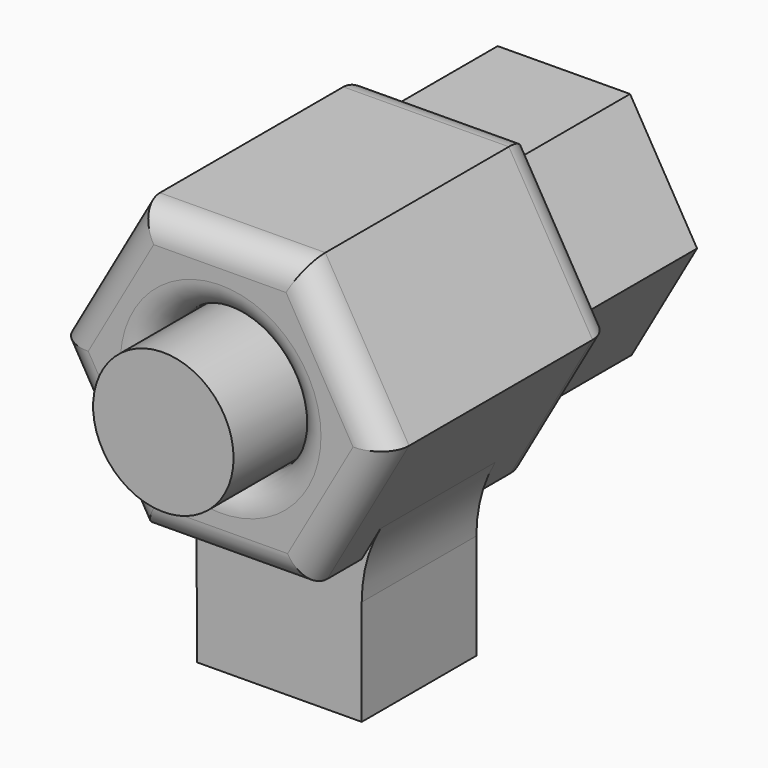
from build123d import *

# Parameters (mm, degrees)
F1_DEPTH    = 25.4
F2_DEPTH    = 12.7
F3_T1_DEPTH = 25.4
F4_R        = 12.7
F5_DEPTH    = 50.801
F6_R        = 5.08
F8_D        = 5.1054
F8_DEPTH    = 16.51
F8_TIP      = 1.5338169022
F9_DEPTH    = 25.4
F10_R       = 12.446
F11_DEPTH   = 12.7


# Not quite as in the source:
# - a fillet or chamfer that OpenCascade refuses, or shapes differently, is made with other operations: its cross-section is extruded or revolved along the edge and cut away or added


with BuildPart() as f1:
    # F0 (on Front) → F1 (new body, symmetric)
    with BuildSketch(Plane.XZ):
        Polygon((14.8365712132, -25.2999898808), (29.3287195589, 0.1988526353), (14.4921483457, 25.4988425161), (-14.8365712132, 25.2999898808), (-29.3287195589, -0.1988526353), (-14.4921483457, -25.4988425161), align=None)
    extrude(amount=F1_DEPTH, both=True)

    # F0 (on Front) → F2 (join, symmetric)
    with BuildSketch(Plane.XZ):
        Polygon((14.8365712132, -50.7005736958), (14.8365712132, -25.2999898808), (-14.4921483457, -25.4988425161), (-14.3199369119, -50.8982587146), align=None)
    extrude(amount=F2_DEPTH, both=True)

    # F3: fillet of radius 25.4 on 6 edges, made by hand

    # F3_s2 → F3_t1 (join)
    with BuildSketch(Plane.XZ.offset(-12.7)):
        with BuildLine():
            ThreePointArc((18.1539258272, -19.463125611), (15.6799102756, -25.5229004766), (14.8365712132, -32.0136942337))
            Line((14.8365712132, -32.0136942337), (14.8365712132, -25.2999898808))
            Line((14.8365712132, -25.2999898808), (18.1539258272, -19.463125611))
        make_face()
        with BuildLine():
            ThreePointArc((-17.9349866772, -19.6279594328), (-15.3560401496, -25.7366108904), (-14.446004431, -32.3045955747))
            Line((-14.446004431, -32.3045955747), (-14.4921483457, -25.4988425161))
            Line((-14.4921483457, -25.4988425161), (-17.9349866772, -19.6279594328))
        make_face()
    extrude(amount=F3_T1_DEPTH)

    # F4 (on face) → F5 (cut, through all)
    with BuildSketch(Plane.XZ.offset(25.4)):
        Circle(F4_R)
    extrude(amount=-F5_DEPTH, mode=Mode.SUBTRACT)

    # F6
    f6_edges = [f1.edges().sort_by_distance(p)[0] for p in [
        (-21.910434, -25.4, -12.848848),
        (-22.082645, -25.4, 12.550569),
        (0.172211, -25.4, -25.399416),
        (-0.172211, -25.4, 25.399416),
        (22.082645, -25.4, -12.550569),
        (21.910434, -25.4, 12.848848),
        (-12.7, -25.4, 0),
        (-21.910434, 25.4, -12.848848),
        (-22.082645, 25.4, 12.550569),
        (0.172211, 25.4, -25.399416),
        (-0.172211, 25.4, 25.399416),
        (22.082645, 25.4, -12.550569),
        (21.910434, 25.4, 12.848848),
        (-12.7, 25.4, 0),
    ]]
    fillet(f6_edges, radius=F6_R)

    # F8
    with Locations(Plane(origin=(0.3444228676, 0, -50.7988323969), x_dir=(0.9999770157, 0, 0.0067799777), z_dir=(0.0067799777, 0, -0.9999770157))):
        with Locations((0, 0)):
            Hole(F8_D / 2, depth=F8_DEPTH)
            with Locations((0, 0, -(F8_DEPTH + F8_TIP / 2))):  # 118° drill point
                Cone(0, F8_D / 2, F8_TIP, mode=Mode.SUBTRACT)


with BuildPart() as f9:
    # F9 (new): a face of the model
    f9_faces = [f1.part.faces().sort_by_distance(p)[0] for p in [
        (-16.9919602561, 25.4, -9.9645268468),
    ]]
    extrude(f9_faces, amount=F9_DEPTH)


with BuildPart() as f11:
    # F10 (on face) → F11 (new body, symmetric)
    with BuildSketch(Plane.XZ.offset(25.4)):
        Circle(F10_R)
    extrude(amount=F11_DEPTH, both=True)


solid = Compound([f1.part, f9.part, f11.part])
